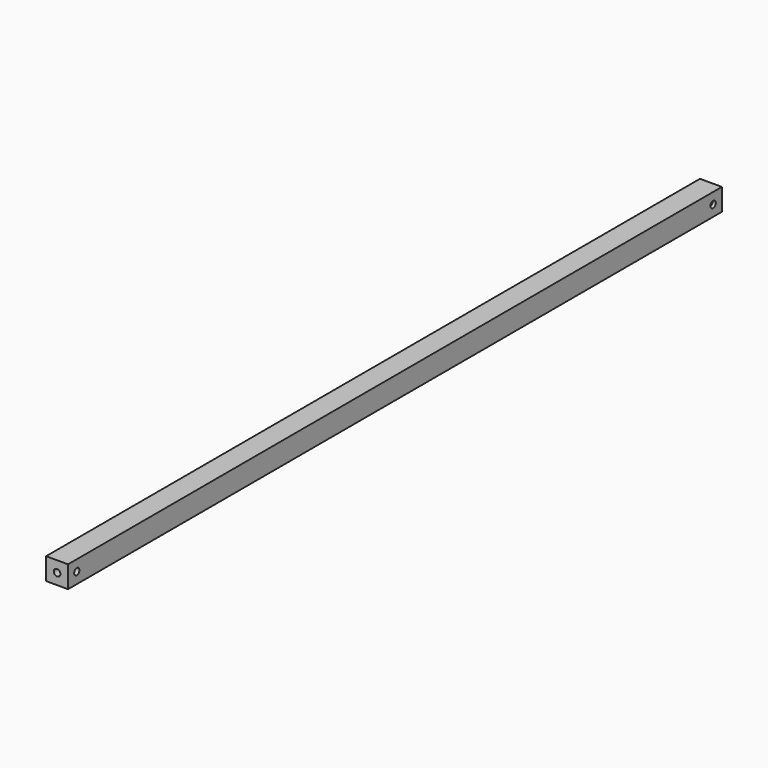
from build123d import *

# Parameters (mm, degrees)
F0_W     = 20
F0_H     = 20
F1_DEPTH = 372.4825
F2_R     = 3
F3_DEPTH = 12
F4_R     = 3
F5_DEPTH = 12
F6_R     = 3
F7_DEPTH = 3
F8_R     = 3
F9_DEPTH = 4


with BuildPart() as f1:
    # F0 (on Front) → F1 (new body, symmetric)
    with BuildSketch(Plane.XZ):
        with Locations((10, 10)):
            Rectangle(F0_W, F0_H)
    extrude(amount=F1_DEPTH, both=True)

    # F2 (on face) → F3 (cut)
    with BuildSketch(Plane.XZ.offset(372.4825)):
        with Locations((10, 10)):
            Circle(F2_R)
    extrude(amount=-F3_DEPTH, mode=Mode.SUBTRACT)

    # F4 (on face) → F5 (cut)
    with BuildSketch(Plane(origin=(0, 372.4825, 0), x_dir=(-1, 0, 0), z_dir=(0, 1, 0))):
        with Locations((-10, 10)):
            Circle(F4_R)
    extrude(amount=-F5_DEPTH, mode=Mode.SUBTRACT)

    # F6 (on face) → F7 (cut)
    with BuildSketch(Plane.YZ.offset(20)):
        with Locations((362.4825, 10)):
            Circle(F6_R)
    extrude(amount=-F7_DEPTH, mode=Mode.SUBTRACT)

    # F8 (on face) → F9 (cut)
    with BuildSketch(Plane.YZ.offset(20)):
        with Locations((-362.4825, 10)):
            Circle(F8_R)
    extrude(amount=-F9_DEPTH, mode=Mode.SUBTRACT)


solid = f1.part
